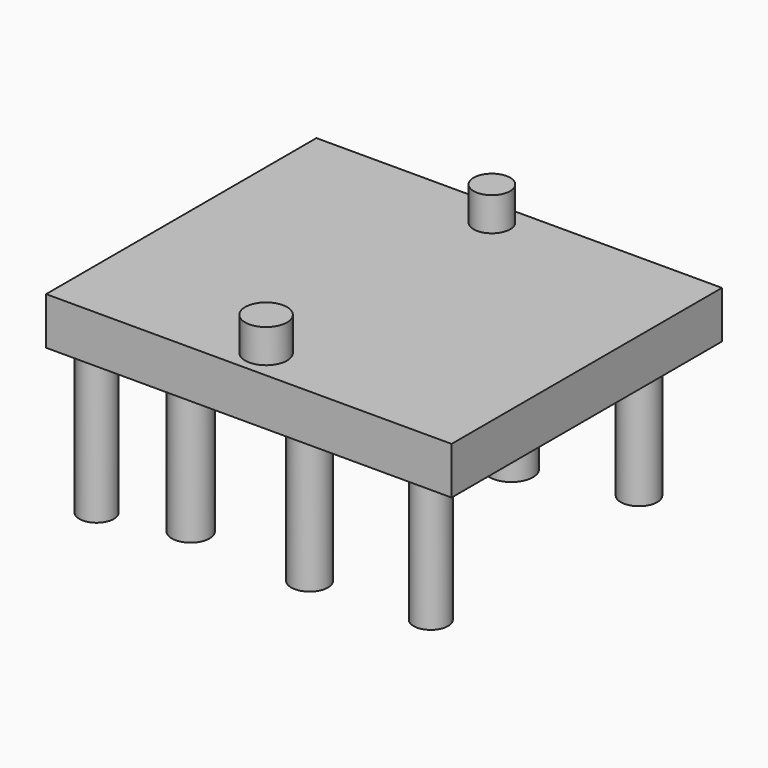
from build123d import *

# Parameters (mm, degrees)
F0_W      = 76.2
F0_H      = 63.5
F1_DEPTH  = 8.87915
F2_R      = 3.2312727432
F3_DEPTH  = 27.64789
F2_R_2    = 3.4736024705
F2_R_3    = 3.4228960701
F2_R_4    = 3.2312730123
F4_DEPTH  = 25.4
F5_R      = 3.9275858197
F5_R_2    = 3.4275613836
F6_DEPTH  = 6.31556
F9_R      = 4.0783648595
F9_R_2    = 3.9191806832
F9_R_3    = 3.5394300608
F9_R_4    = 3.4524766022
F10_DEPTH = 25.4


# Not quite as in the source:
# - the program builds the solid bodies; features that only make, move or delete a surface that nothing else refers to are left out


with BuildPart() as f1:
    # F0 (on Top) → F1 (new body)
    with BuildSketch(Plane.XY):
        with Locations((-14.3929980695, -5.2504202625)):
            Rectangle(F0_W, F0_H)
    extrude(amount=F1_DEPTH)

    # F2 (on face) → F3 (join)
    with BuildSketch(Plane(origin=(0, 0, 0), x_dir=(1, 0, 0), z_dir=(0, 0, -1))):
        with Locations((-47.1578612924, 31.7992158234)):
            Circle(F2_R)
    extrude(amount=F3_DEPTH)

    # F2 (on face) → F4 (join)
    with BuildSketch(Plane(origin=(0, 0, 0), x_dir=(1, 0, 0), z_dir=(0, 0, -1))):
        with Locations((-47.1578612924, 31.7992158234)):
            Circle(F2_R)
        with Locations((-47.1578612924, -17.4867473543)):
            Circle(F2_R_2)
        with Locations((14.2814768478, -18.8030768186)):
            Circle(F2_R_3)
        with Locations((15.0982076302, 31.1281010509)):
            Circle(F2_R_4)
    extrude(amount=F4_DEPTH)

    # F5 (on face) → F6 (join)
    with BuildSketch(Plane.XY.offset(8.87915)):
        with Locations((-15.6099880114, -31.4252711833)):
            Circle(F5_R)
        with Locations((-15.6099880114, 21.6196272522)):
            Circle(F5_R_2)
    extrude(amount=F6_DEPTH)

    # F9 (on face) → F10 (join)
    with BuildSketch(Plane(origin=(0, 0, 0), x_dir=(1, 0, 0), z_dir=(0, 0, -1))):
        with Locations((-5.5510420352, -13.5985026136)):
            Circle(F9_R)
        with Locations((-28.7904683501, -13.2877733558)):
            Circle(F9_R_2)
        with Locations((-29.9201626331, 31.2515720725)):
            Circle(F9_R_3)
        with Locations((-6.5234871581, 32.5696654618)):
            Circle(F9_R_4)
    extrude(amount=F10_DEPTH)


solid = f1.part
